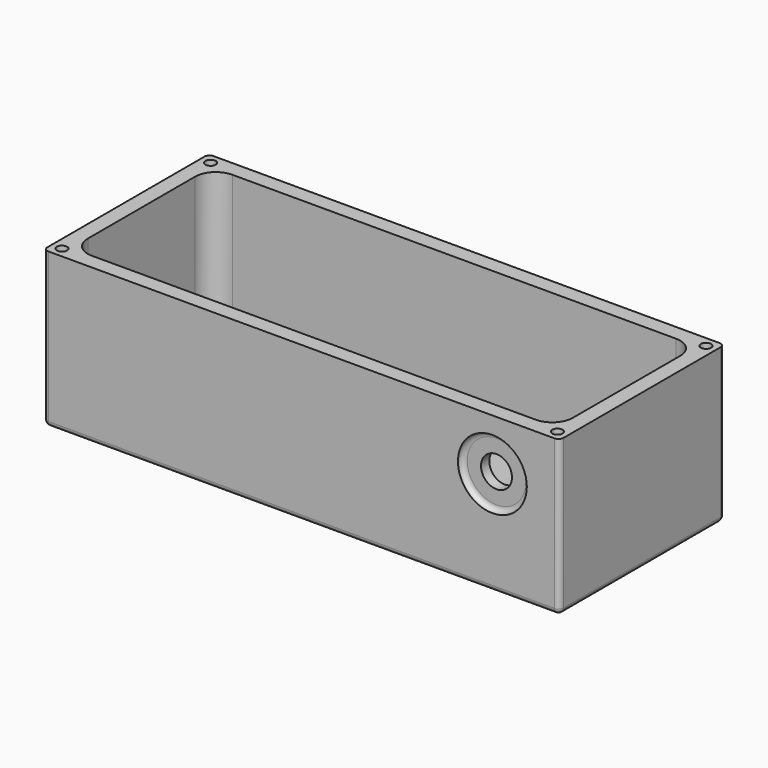
from build123d import *

# Parameters (mm, degrees)
F0_W      = 100
F0_H      = 40
F0_R      = 1.5
F1_DEPTH  = 30
F2_W      = 94
F2_H      = 34
F2_R      = 1
F3_DEPTH  = 27
F4_R      = 3
F5_DEPTH  = 5
F6_R      = 1
F7_R      = 4
F8_R      = 4
F9_R      = 6.6732690133
F10_DEPTH = 1
F11_R     = 0.99999


# Not quite as in the source:
# - a fillet or chamfer is up to 0.001 mm smaller than in the source, because OpenCascade refuses the exact size


with BuildPart() as f1:
    # F0 (on Top) → F1 (new body)
    with BuildSketch(Plane.XY):
        with Locations((-4.7806398869, -4.191e-06)):
            Rectangle(F0_W, F0_H)
        with Locations((-21.7806398869, 0)):
            Circle(F0_R, mode=Mode.SUBTRACT)
        with Locations((12.2193601131, 0)):
            Circle(F0_R, mode=Mode.SUBTRACT)
    extrude(amount=F1_DEPTH)

    # F2 (on face) → F3 (cut)
    with BuildSketch(Plane.XY.offset(30)):
        with Locations((-4.7806398869, -4.191e-06)):
            Rectangle(F2_W, F2_H)
        with Locations((-52.7806398869, 17.999995809)):
            Circle(F2_R)
        with Locations((-52.7806398869, -18.000004191)):
            Circle(F2_R)
        with Locations((43.2193601131, 17.999995809)):
            Circle(F2_R)
        with Locations((43.2193601131, -18.000004191)):
            Circle(F2_R)
    extrude(amount=-F3_DEPTH, mode=Mode.SUBTRACT)

    # F4 (on face) → F5 (cut)
    with BuildSketch(Plane.XZ.offset(20.000004191)):
        with Locations((32.2193601131, 20)):
            Circle(F4_R)
    extrude(amount=-F5_DEPTH, mode=Mode.SUBTRACT)

    # F6
    f6_edges = [f1.edges().sort_by_distance(p)[0] for p in [
        (45.21936, 19.999996, 15),
        (-4.78064, 19.999996, 0),
        (45.21936, -4e-06, 0),
        (45.21936, -20.000004, 15),
        (-4.78064, -20.000004, 0),
        (-54.78064, -4e-06, 0),
        (-54.78064, 19.999996, 15),
        (-54.78064, -20.000004, 15),
    ]]
    fillet(f6_edges, radius=F6_R)

    # F7
    f7_edges = [f1.edges().sort_by_distance(p)[0] for p in [
        (42.21936, 16.999996, 16.5),
        (-51.78064, 16.999996, 16.5),
        (-51.78064, -17.000004, 16.5),
        (42.21936, -17.000004, 16.5),
    ]]
    fillet(f7_edges, radius=F7_R)

    # F8
    f8_edges = [f1.edges().sort_by_distance(p)[0] for p in [
        (-4.78064, 16.999996, 3),
    ]]
    fillet(f8_edges, radius=F8_R)

    # F9 (on face) → F10 (cut)
    with BuildSketch(Plane.XZ.offset(20.000004191)):
        with Locations((32.2193601131, 20)):
            Circle(F9_R)
    extrude(amount=-F10_DEPTH, mode=Mode.SUBTRACT)

    # F11 (radius 1 in the source; OpenCascade refuses exactly that, so slightly less here)
    f11_edges = [f1.edges().sort_by_distance(p)[0] for p in [
        (25.546091, -19.000004, 20),
    ]]
    fillet(f11_edges, radius=F11_R)


solid = f1.part
